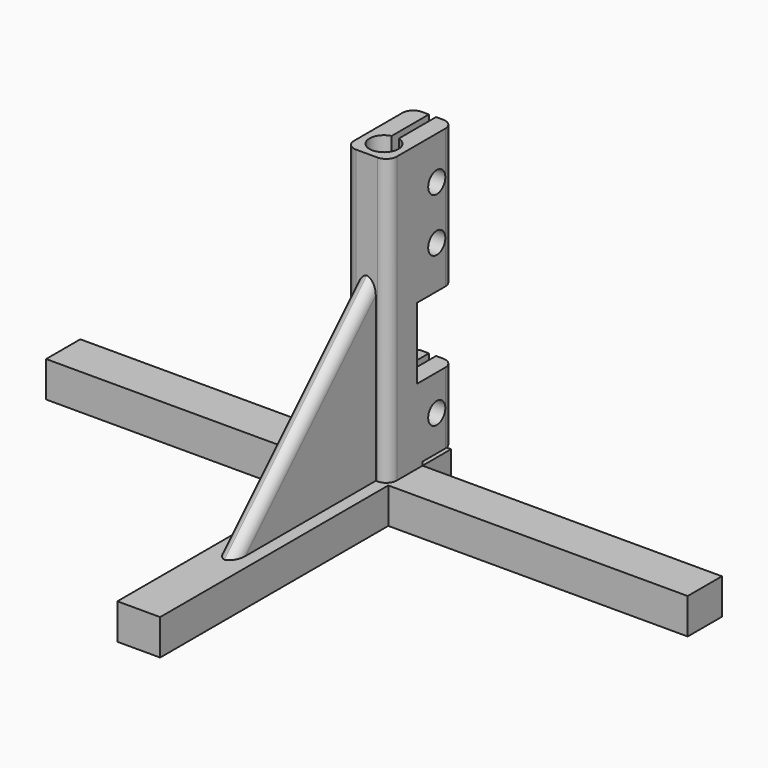
from build123d import *

# Parameters (mm, degrees)
F1_DEPTH      = 10
F3_W          = 12
F3_H          = 23
F3_R          = 4.05
F4_DEPTH      = 80
F5_W          = 2
F5_H          = 39.0547718853
F6_DEPTH      = 80
F7_W          = 11
F7_H          = 1
F7_W_2        = 13
F7_H_2        = 20
F7_R          = 3
F8_DEPTH      = 25
F10_DEPTH     = 2.5
F11_T1_DEPTH  = 87.5
F11_T3_DEPTH  = 54
F11_T5_DEPTH  = 27.5
F11_T10_DEPTH = 85.7106781187
F11_T16_DEPTH = 85.7106781187


# Not quite as in the source:
# - a fillet or chamfer that OpenCascade refuses, or shapes differently, is made with other operations: its cross-section is extruded or revolved along the edge and cut away or added


with BuildPart() as f1:
    # F0 (on Top) → F1 (new body)
    with BuildSketch(Plane.XY):
        Polygon((6, 22), (0, 22), (-6, 22), (-6, 12), (-90, 12), (-90, 0), (-6, 0), (-6, -80), (6, -80), (6, 0), (90, 0), (90, 12), (6, 12), align=None)
    extrude(amount=F1_DEPTH)

    # F3 (on face) → F4 (join)
    with BuildSketch(Plane.XY.offset(10)):
        with Locations((0, 11.5)):
            Rectangle(F3_W, F3_H)
        with Locations((0, 6)):
            Circle(F3_R, mode=Mode.SUBTRACT)
    extrude(amount=F4_DEPTH)

    # F5 (on face) → F6 (cut, through all)
    with BuildSketch(Plane.XY.offset(10)):
        with Locations((0, 25.7887821645)):
            Rectangle(F5_W, F5_H)
    extrude(amount=F6_DEPTH, mode=Mode.SUBTRACT)

    # F7 (on face) → F8 (cut)
    with BuildSketch(Plane(origin=(-6, 0, 0), x_dir=(0, -1, 0), z_dir=(-1, 0, 0))):
        with Locations((-17.5, 10.5)):
            Rectangle(F7_W, F7_H)
        with Locations((-16.5, 41)):
            Rectangle(F7_W_2, F7_H_2)
        with Locations((-17, 21)):
            Circle(F7_R)
        with Locations((-17, 78)):
            Circle(F7_R)
        with Locations((-17, 63)):
            Circle(F7_R)
    extrude(amount=-F8_DEPTH, mode=Mode.SUBTRACT)

    # F9 (on Right) → F10 (join, symmetric)
    with BuildSketch(Plane.YZ):
        Polygon((0, 10), (0, 60), (-50, 10), align=None)
    extrude(amount=F10_DEPTH, both=True)

    # F11: fillet of radius 3 on 8 edges, made by hand

    # F11_s2 → F11_t1 (cut)
    with BuildSketch(Plane.XY.offset(10)):
        with BuildLine():
            ThreePointArc((-6, 3), (-5.1213203436, 0.8786796564), (-3, 0))
            Line((-3, 0), (-6, 0))
            Line((-6, 0), (-6, 3))
        make_face()
        with BuildLine():
            ThreePointArc((6, 3), (5.1213203436, 0.8786796564), (3, 0))
            Line((3, 0), (6, 0))
            Line((6, 0), (6, 3))
        make_face()
    extrude(amount=F11_T1_DEPTH, mode=Mode.SUBTRACT)

    # F11_s4 → F11_t3 (cut)
    with BuildSketch(Plane.XY.offset(43.5)):
        with BuildLine():
            ThreePointArc((-3, 23), (-5.1213203436, 22.1213203436), (-6, 20))
            Line((-6, 20), (-6, 23))
            Line((-6, 23), (-3, 23))
        make_face()
        with BuildLine():
            ThreePointArc((6, 20), (5.1213203436, 22.1213203436), (3, 23))
            Line((3, 23), (6, 23))
            Line((6, 23), (6, 20))
        make_face()
    extrude(amount=F11_T3_DEPTH, mode=Mode.SUBTRACT)

    # F11_s6 → F11_t5 (cut)
    with BuildSketch(Plane.XY.offset(11)):
        with BuildLine():
            ThreePointArc((6, 20), (5.1213203436, 22.1213203436), (3, 23))
            Line((3, 23), (6, 23))
            Line((6, 23), (6, 20))
        make_face()
        with BuildLine():
            ThreePointArc((-3, 23), (-5.1213203436, 22.1213203436), (-6, 20))
            Line((-6, 20), (-6, 23))
            Line((-6, 23), (-3, 23))
        make_face()
    extrude(amount=F11_T5_DEPTH, mode=Mode.SUBTRACT)


with BuildPart() as f11_tool8:
    # F11_s9 → F11_t10 (new body)
    with BuildSketch(Plane(origin=(0, 35.3033008589, 35.3033008589), x_dir=(1, 0, 0), z_dir=(0, -0.7071067812, -0.7071067812))):
        with BuildLine():
            ThreePointArc((-2.5, 39.4264068712), (-1.6213203436, 41.5477272148), (0.5, 42.4264068712))
            Line((0.5, 42.4264068712), (-2.5, 42.4264068712))
            Line((-2.5, 42.4264068712), (-2.5, 39.4264068712))
        make_face()
    extrude(amount=F11_T10_DEPTH)

    split(bisect_by=Plane.XY.offset(10), keep=Keep.TOP)

    split(bisect_by=Plane.XZ, keep=Keep.TOP)


with BuildPart() as f1_1:
    add(f1.part)

    # F11_t7: cut F11_tool8
    add(f11_tool8.part, mode=Mode.SUBTRACT)


with BuildPart() as f11_tool14:
    # F11_s15 → F11_t16 (new body)
    with BuildSketch(Plane(origin=(0, 35.3033008589, 35.3033008589), x_dir=(1, 0, 0), z_dir=(0, -0.7071067812, -0.7071067812))):
        with BuildLine():
            ThreePointArc((-0.5, 42.4264068712), (1.6213203436, 41.5477272148), (2.5, 39.4264068712))
            Line((2.5, 39.4264068712), (2.5, 42.4264068712))
            Line((2.5, 42.4264068712), (-0.5, 42.4264068712))
        make_face()
    extrude(amount=F11_T16_DEPTH)

    split(bisect_by=Plane.XY.offset(10), keep=Keep.TOP)

    split(bisect_by=Plane.XZ, keep=Keep.TOP)


with BuildPart() as f1_2:
    add(f1_1.part)

    # F11_t13: cut F11_tool14
    add(f11_tool14.part, mode=Mode.SUBTRACT)


solid = f1_2.part
